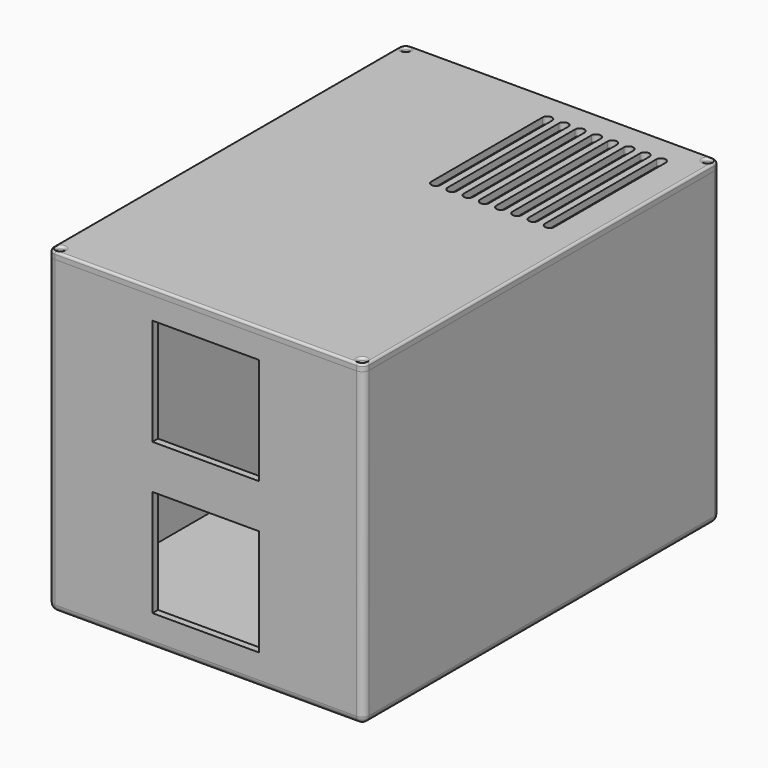
from build123d import *

# Parameters (mm, degrees)
F0_W          = 136
F0_H          = 192
F1_DEPTH      = 4
F2_DEPTH      = 134
F3_W          = 46
F3_H          = 46
F4_DEPTH      = 25
F5_W          = 84
F5_H          = 10
F6_DEPTH      = 20
F8_DEPTH      = 10
F9_W          = 10
F9_H          = 107
F10_DEPTH     = 10
F11_R         = 1.5
F12_DEPTH     = 10
F13_W         = 10
F13_H         = 10
F13_W_2       = 28
F13_H_2       = 68
F13_W_3       = 19
F13_R         = 1.6
F14_DEPTH     = 25
F15_R         = 3
F16_R         = 3
F17_R         = 3
F19_W         = 66
F19_H         = 126
F19_W_2       = 46
F19_H_2       = 46
F20_DEPTH     = 10
F21_SIZE      = 1
F23_R         = 1.5
F24_DEPTH     = 3
F25_T1_DEPTH  = 186
F25_T3_DEPTH  = 130
F25_T6_ANGLE  = 90
F25_T8_ANGLE  = 90
F25_T10_ANGLE = 90
F25_T12_ANGLE = 90
F27_DEPTH     = 25
F28_W         = 2.2
F28_H         = 59
F28_H_2       = 5
F29_DEPTH     = 97


# Not quite as in the source:
# - a fillet or chamfer that OpenCascade refuses, or shapes differently, is made with other operations: its cross-section is extruded or revolved along the edge and cut away or added


with BuildPart() as f1:
    # F0 (on Top) → F1 (new body)
    with BuildSketch(Plane.XY):
        Rectangle(F0_W, F0_H)
        with BuildLine():
            ThreePointArc((65, -88), (61.4644660941, -89.4644660941), (60, -93))
            Line((60, -93), (-60, -93))
            ThreePointArc((-60, -93), (-61.4644660941, -89.4644660941), (-65, -88))
            Line((-65, -88), (-65, 88))
            ThreePointArc((-65, 88), (-61.4644660941, 89.4644660941), (-60, 93))
            Line((-60, 93), (60, 93))
            ThreePointArc((60, 93), (61.4644660941, 89.4644660941), (65, 88))
            Line((65, 88), (65, -88))
        make_face(mode=Mode.SUBTRACT)
        with BuildLine():
            Line((-60, -93), (60, -93))
            ThreePointArc((60, -93), (61.4644660941, -89.4644660941), (65, -88))
            Line((65, -88), (65, 88))
            ThreePointArc((65, 88), (61.4644660941, 89.4644660941), (60, 93))
            Line((60, 93), (-60, 93))
            ThreePointArc((-60, 93), (-61.4644660941, 89.4644660941), (-65, 88))
            Line((-65, 88), (-65, -88))
            ThreePointArc((-65, -88), (-61.4644660941, -89.4644660941), (-60, -93))
        make_face()
    extrude(amount=F1_DEPTH)

    # F0 (on Top) → F2 (join)
    with BuildSketch(Plane.XY):
        Rectangle(F0_W, F0_H)
        with BuildLine():
            ThreePointArc((65, -88), (61.4644660941, -89.4644660941), (60, -93))
            Line((60, -93), (-60, -93))
            ThreePointArc((-60, -93), (-61.4644660941, -89.4644660941), (-65, -88))
            Line((-65, -88), (-65, 88))
            ThreePointArc((-65, 88), (-61.4644660941, 89.4644660941), (-60, 93))
            Line((-60, 93), (60, 93))
            ThreePointArc((60, 93), (61.4644660941, 89.4644660941), (65, 88))
            Line((65, 88), (65, -88))
        make_face(mode=Mode.SUBTRACT)
    extrude(amount=F2_DEPTH)

    # F3 (on face) → F4 (cut)
    with BuildSketch(Plane.XZ.offset(96)):
        with Locations((0, 101.5)):
            Rectangle(F3_W, F3_H)
        with Locations((0, 36.5)):
            Rectangle(F3_W, F3_H)
    extrude(amount=-F4_DEPTH, mode=Mode.SUBTRACT)

    # F5 (on face) → F6 (join)
    with BuildSketch(Plane.XY.offset(4)):
        with Locations((-23, 78)):
            Rectangle(F5_W, F5_H)
    extrude(amount=F6_DEPTH)

    # F7 (on face) → F8 (cut)
    with BuildSketch(Plane.XZ.offset(-73)):
        Polygon((-28, 14), (-18, 14), (9, 14), (9, 4), (19, 4), (19, 24), (19, 33.6412377656), (-55, 33.6412377656), (-65, 33.6412377656), (-65, 24), (-65, 14), (-55, 14), align=None)
    extrude(amount=-F8_DEPTH, mode=Mode.SUBTRACT)

    # F9 (on face) → F10 (join)
    with BuildSketch(Plane(origin=(65, 0, 0), x_dir=(0, -1, 0), z_dir=(-1, 0, 0))):
        with Locations((-78, 57.5)):
            Rectangle(F9_W, F9_H)
        with Locations((-14, 57.5)):
            Rectangle(F9_W, F9_H)
    extrude(amount=F10_DEPTH)

    # F11 (on face) → F12 (cut)
    with BuildSketch(Plane.XY.offset(134)):
        with Locations((65, 93)):
            Circle(F11_R)
        with Locations((-65, 93)):
            Circle(F11_R)
        with Locations((65, -93)):
            Circle(F11_R)
        with Locations((-65, -93)):
            Circle(F11_R)
    extrude(amount=-F12_DEPTH, mode=Mode.SUBTRACT)

    # F13 (on face) → F14 (cut)
    with BuildSketch(Plane(origin=(0, 96, 0), x_dir=(-1, 0, 0), z_dir=(0, 1, 0))):
        with Locations((-40, 129)):
            Rectangle(F13_W, F13_H)
        with Locations((42, 48)):
            Rectangle(F13_W_2, F13_H_2)
        with Locations((4, 48)):
            Rectangle(F13_W_2, F13_H_2)
        with Locations((-31.5, 47.8000001609)):
            Rectangle(F13_W_3, F13_H)
        with Locations((-44, 47.8000001609)):
            Circle(F13_R)
        with Locations((-19, 47.8000001609)):
            Circle(F13_R)
        with Locations((-44, 69.5999908447)):
            Circle(F13_R)
        with Locations((-31.5, 69.5999908447)):
            Rectangle(F13_W_3, F13_H)
        with Locations((-19, 69.5999908447)):
            Circle(F13_R)
    extrude(amount=-F14_DEPTH, mode=Mode.SUBTRACT)

    # F15
    f15_edges = [f1.edges().sort_by_distance(p)[0] for p in [
        (-68, -96, 67),
        (68, -96, 67),
        (68, 96, 67),
        (-68, 96, 67),
    ]]
    fillet(f15_edges, radius=F15_R)

    # F16
    f16_edges = [f1.edges().sort_by_distance(p)[0] for p in [
        (0, -96, 0),
    ]]
    fillet(f16_edges, radius=F16_R)

    # F17
    f17_edges = [f1.edges().sort_by_distance(p)[0] for p in [
        (45, 94.5, 124),
        (35, 94.5, 124),
    ]]
    fillet(f17_edges, radius=F17_R)

    # F28 (on face) → F29 (cut)
    with BuildSketch(Plane.XY.offset(111)):
        with Locations((60, 48.5)):
            Rectangle(F28_W, F28_H)
        with Locations((60, 16.5)):
            Rectangle(F28_W, F28_H_2)
    extrude(amount=-F29_DEPTH, mode=Mode.SUBTRACT)


with BuildPart() as f20:
    # F19 (on offset) → F20 (new body)
    with BuildSketch(Plane(origin=(0, -23, 0), x_dir=(-1, 0, 0), z_dir=(0, 1, 0))):
        with Locations((0, 66.5)):
            Rectangle(F19_W, F19_H)
        with Locations((0, 36.5)):
            Rectangle(F19_W_2, F19_H_2, mode=Mode.SUBTRACT)
        with Locations((0, 101.5)):
            Rectangle(F19_W_2, F19_H_2, mode=Mode.SUBTRACT)
    extrude(amount=F20_DEPTH)

    # F21
    f21_edges = [f20.edges().sort_by_distance(p)[0] for p in [
        (-33, -23, 66.5),
        (0, -23, 129.5),
        (33, -23, 66.5),
        (0, -23, 3.5),
        (23, -23, 36.5),
        (0, -23, 59.5),
        (-23, -23, 36.5),
        (0, -23, 13.5),
        (23, -23, 101.5),
        (0, -23, 124.5),
        (-23, -23, 101.5),
        (0, -23, 78.5),
        (-33, -13, 66.5),
        (0, -13, 129.5),
        (33, -13, 66.5),
        (0, -13, 3.5),
        (23, -13, 36.5),
        (0, -13, 59.5),
        (-23, -13, 36.5),
        (0, -13, 13.5),
        (23, -13, 101.5),
        (0, -13, 124.5),
        (-23, -13, 101.5),
        (0, -13, 78.5),
    ]]
    chamfer(f21_edges, length=F21_SIZE)


with BuildPart() as f24:
    # F23 (on offset) → F24 (new body)
    with BuildSketch(Plane.XY.offset(134)):
        with BuildLine():
            ThreePointArc((65, -96), (67.1213203436, -95.1213203436), (68, -93))
            Line((68, -93), (68, 93))
            ThreePointArc((68, 93), (67.1213203436, 95.1213203436), (65, 96))
            Line((65, 96), (-65, 96))
            ThreePointArc((-65, 96), (-67.1213203436, 95.1213203436), (-68, 93))
            Line((-68, 93), (-68, -93))
            ThreePointArc((-68, -93), (-67.1213203436, -95.1213203436), (-65, -96))
            Line((-65, -96), (65, -96))
        make_face()
        with Locations((-65, -93)):
            Circle(F23_R, mode=Mode.SUBTRACT)
        with Locations((65, -93)):
            Circle(F23_R, mode=Mode.SUBTRACT)
        with Locations((-65, 93)):
            Circle(F23_R, mode=Mode.SUBTRACT)
        with BuildLine():
            Line((-60, 93), (60, 93))
            ThreePointArc((60, 93), (61.4644660941, 89.4644660941), (65, 88))
            Line((65, 88), (65, -88))
            ThreePointArc((65, -88), (61.4644660941, -89.4644660941), (60, -93))
            Line((60, -93), (-60, -93))
            ThreePointArc((-60, -93), (-61.4644660941, -89.4644660941), (-65, -88))
            Line((-65, -88), (-65, 88))
            ThreePointArc((-65, 88), (-61.4644660941, 89.4644660941), (-60, 93))
        make_face(mode=Mode.SUBTRACT)
        with Locations((65, 93)):
            Circle(F23_R, mode=Mode.SUBTRACT)
        with BuildLine():
            ThreePointArc((65, 88), (61.4644660941, 89.4644660941), (60, 93))
            Line((60, 93), (-60, 93))
            ThreePointArc((-60, 93), (-61.4644660941, 89.4644660941), (-65, 88))
            Line((-65, 88), (-65, -88))
            ThreePointArc((-65, -88), (-61.4644660941, -89.4644660941), (-60, -93))
            Line((-60, -93), (60, -93))
            ThreePointArc((60, -93), (61.4644660941, -89.4644660941), (65, -88))
            Line((65, -88), (65, 88))
        make_face()
        with BuildLine():
            Line((64, 87.0839202169), (64, -87.0839202169))
            ThreePointArc((64, -87.0839202169), (60.7573593129, -88.7573593129), (59.0839202169, -92))
            Line((59.0839202169, -92), (-59.0839202169, -92))
            ThreePointArc((-59.0839202169, -92), (-60.7573593129, -88.7573593129), (-64, -87.0839202169))
            Line((-64, -87.0839202169), (-64, 87.0839202169))
            ThreePointArc((-64, 87.0839202169), (-60.7573593129, 88.7573593129), (-59.0839202169, 92))
            Line((-59.0839202169, 92), (59.0839202169, 92))
            ThreePointArc((59.0839202169, 92), (60.7573593129, 88.7573593129), (64, 87.0839202169))
        make_face(mode=Mode.SUBTRACT)
        with BuildLine():
            ThreePointArc((59.0839202169, -92), (60.7573593129, -88.7573593129), (64, -87.0839202169))
            Line((64, -87.0839202169), (64, 87.0839202169))
            ThreePointArc((64, 87.0839202169), (60.7573593129, 88.7573593129), (59.0839202169, 92))
            Line((59.0839202169, 92), (-59.0839202169, 92))
            ThreePointArc((-59.0839202169, 92), (-60.7573593129, 88.7573593129), (-64, 87.0839202169))
            Line((-64, 87.0839202169), (-64, -87.0839202169))
            ThreePointArc((-64, -87.0839202169), (-60.7573593129, -88.7573593129), (-59.0839202169, -92))
            Line((-59.0839202169, -92), (59.0839202169, -92))
        make_face()
    extrude(amount=F24_DEPTH)

    # F25: fillet of radius 1 on 12 edges, made by hand

    # F25_s2 → F25_t1 (cut)
    with BuildSketch(Plane.XZ.offset(-93)):
        with BuildLine():
            ThreePointArc((68, 136), (67.7071067812, 136.7071067812), (67, 137))
            Line((67, 137), (68, 137))
            Line((68, 137), (68, 136))
        make_face()
        with BuildLine():
            ThreePointArc((-68, 136), (-67.7071067812, 136.7071067812), (-67, 137))
            Line((-67, 137), (-68, 137))
            Line((-68, 137), (-68, 136))
        make_face()
    extrude(amount=F25_T1_DEPTH, mode=Mode.SUBTRACT)

    # F25_s4 → F25_t3 (cut)
    with BuildSketch(Plane.YZ.offset(-65)):
        with BuildLine():
            ThreePointArc((96, 136), (95.7071067812, 136.7071067812), (95, 137))
            Line((95, 137), (96, 137))
            Line((96, 137), (96, 136))
        make_face()
        with BuildLine():
            ThreePointArc((-96, 136), (-95.7071067812, 136.7071067812), (-95, 137))
            Line((-95, 137), (-96, 137))
            Line((-96, 137), (-96, 136))
        make_face()
    extrude(amount=F25_T3_DEPTH, mode=Mode.SUBTRACT)

    # F25_s5 → F25_t6 (revolve, cut)
    with BuildSketch(Plane.YZ.offset(65)):
        with BuildLine():
            ThreePointArc((-96, 136), (-95.7071067812, 136.7071067812), (-95, 137))
            Line((-95, 137), (-96, 137))
            Line((-96, 137), (-96, 136))
        make_face()
    revolve(axis=Axis((65, -93, 137), (0, 0, 1)), revolution_arc=F25_T6_ANGLE, mode=Mode.SUBTRACT)

    # F25_s7 → F25_t8 (revolve, cut)
    with BuildSketch(Plane.XZ.offset(-93)):
        with BuildLine():
            ThreePointArc((68, 136), (67.7071067812, 136.7071067812), (67, 137))
            Line((67, 137), (68, 137))
            Line((68, 137), (68, 136))
        make_face()
    revolve(axis=Axis((65, 93, 137), (0, 0, 1)), revolution_arc=F25_T8_ANGLE, mode=Mode.SUBTRACT)

    # F25_s9 → F25_t10 (revolve, cut)
    with BuildSketch(Plane.YZ.offset(-65)):
        with BuildLine():
            ThreePointArc((96, 136), (95.7071067812, 136.7071067812), (95, 137))
            Line((95, 137), (96, 137))
            Line((96, 137), (96, 136))
        make_face()
    revolve(axis=Axis((-65, 93, 137), (0, 0, 1)), revolution_arc=F25_T10_ANGLE, mode=Mode.SUBTRACT)

    # F25_s11 → F25_t12 (revolve, cut)
    with BuildSketch(Plane.XZ.offset(93)):
        with BuildLine():
            ThreePointArc((-68, 136), (-67.7071067812, 136.7071067812), (-67, 137))
            Line((-67, 137), (-68, 137))
            Line((-68, 137), (-68, 136))
        make_face()
    revolve(axis=Axis((-65, -93, 137), (0, 0, 1)), revolution_arc=F25_T12_ANGLE, mode=Mode.SUBTRACT)

    # F25_s13 → F25_t14 (revolve, cut)
    with BuildSketch(Plane.XZ.offset(93)):
        with BuildLine():
            ThreePointArc((-63.5, 136), (-63.2071067812, 136.7071067812), (-62.5, 137))
            Line((-62.5, 137), (-63.5, 137))
            Line((-63.5, 137), (-63.5, 136))
        make_face()
    revolve(axis=Axis((-65, -93, 137), (0, 0, 1)), mode=Mode.SUBTRACT)

    # F25_s15 → F25_t16 (revolve, cut)
    with BuildSketch(Plane.XZ.offset(93)):
        with BuildLine():
            ThreePointArc((66.5, 136), (66.7928932188, 136.7071067812), (67.5, 137))
            Line((67.5, 137), (66.5, 137))
            Line((66.5, 137), (66.5, 136))
        make_face()
    revolve(axis=Axis((65, -93, 137), (0, 0, 1)), mode=Mode.SUBTRACT)

    # F25_s17 → F25_t18 (revolve, cut)
    with BuildSketch(Plane.XZ.offset(-93)):
        with BuildLine():
            ThreePointArc((-63.5, 136), (-63.2071067812, 136.7071067812), (-62.5, 137))
            Line((-62.5, 137), (-63.5, 137))
            Line((-63.5, 137), (-63.5, 136))
        make_face()
    revolve(axis=Axis((-65, 93, 137), (0, 0, 1)), mode=Mode.SUBTRACT)

    # F25_s19 → F25_t20 (revolve, cut)
    with BuildSketch(Plane.XZ.offset(-93)):
        with BuildLine():
            ThreePointArc((66.5, 136), (66.7928932188, 136.7071067812), (67.5, 137))
            Line((67.5, 137), (66.5, 137))
            Line((66.5, 137), (66.5, 136))
        make_face()
    revolve(axis=Axis((65, 93, 137), (0, 0, 1)), mode=Mode.SUBTRACT)

    # F26 (on face) → F27 (cut)
    with BuildSketch(Plane.XY.offset(137)):
        with BuildLine():
            ThreePointArc((6, 83), (4, 85), (2, 83))
            Line((2, 83), (2, 23))
            ThreePointArc((2, 23), (4, 21), (6, 23))
            Line((6, 23), (6, 83))
        make_face()
        with BuildLine():
            Line((13, 23), (13, 83))
            ThreePointArc((13, 83), (11, 85), (9, 83))
            Line((9, 83), (9, 23))
            ThreePointArc((9, 23), (11, 21), (13, 23))
        make_face()
        with BuildLine():
            Line((20, 23), (20, 83))
            ThreePointArc((20, 83), (18, 85), (16, 83))
            Line((16, 83), (16, 23))
            ThreePointArc((16, 23), (18, 21), (20, 23))
        make_face()
        with BuildLine():
            Line((27, 23), (27, 83))
            ThreePointArc((27, 83), (25, 85), (23, 83))
            Line((23, 83), (23, 23))
            ThreePointArc((23, 23), (25, 21), (27, 23))
        make_face()
        with BuildLine():
            Line((34, 23), (34, 83))
            ThreePointArc((34, 83), (32, 85), (30, 83))
            Line((30, 83), (30, 23))
            ThreePointArc((30, 23), (32, 21), (34, 23))
        make_face()
        with BuildLine():
            Line((41, 23), (41, 83))
            ThreePointArc((41, 83), (39, 85), (37, 83))
            Line((37, 83), (37, 23))
            ThreePointArc((37, 23), (39, 21), (41, 23))
        make_face()
        with BuildLine():
            Line((48, 23), (48, 83))
            ThreePointArc((48, 83), (46, 85), (44, 83))
            Line((44, 83), (44, 23))
            ThreePointArc((44, 23), (46, 21), (48, 23))
        make_face()
        with BuildLine():
            Line((55, 23), (55, 83))
            ThreePointArc((55, 83), (53, 85), (51, 83))
            Line((51, 83), (51, 23))
            ThreePointArc((51, 23), (53, 21), (55, 23))
        make_face()
    extrude(amount=-F27_DEPTH, mode=Mode.SUBTRACT)


solid = Compound([f1.part, f20.part, f24.part])
